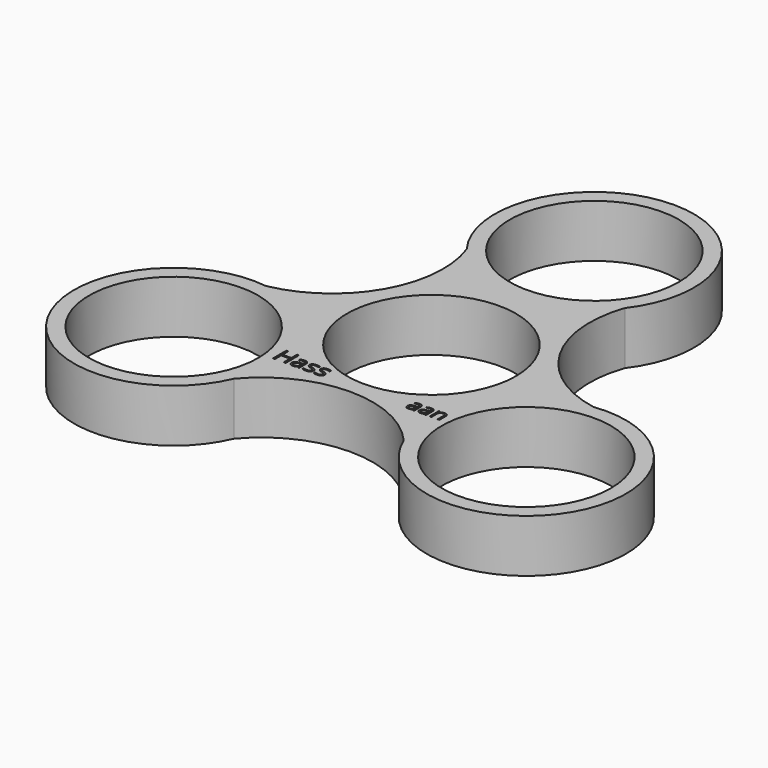
from build123d import *

# Parameters (mm, degrees)
F0_R         = 11.2
F1_DEPTH     = 7
F2_TEXT_SIZE = 3.0873436845
F3_DEPTH     = 0.51
F4_TEXT_SIZE = 2.8406800185
F5_DEPTH     = 0.64


# Not quite as in the source:
# - Text() gives the source's letters only with a copy of the font that has no kerning and outlines rounded to 1/6400 em; it was checked with that copy


with BuildPart() as f1:
    # F0 (on Top) → F1 (new body)
    with BuildSketch(Plane.XY):
        with BuildLine():
            ThreePointArc((21.7602352684, -0.3790794713), (11.6629101979, 6.6669216362), (10.4657940357, 18.9212685418))
            ThreePointArc((10.4657940357, 18.9212685418), (0.0710858988, 40.165152914), (-10.551825182, 19.0344562705))
            ThreePointArc((-10.551825182, 19.0344562705), (-11.605178601, 6.7669156953), (-21.6191962469, -0.3969907652))
            ThreePointArc((-21.6191962469, -0.3969907652), (-34.8195857199, -20.0210142628), (-11.2084100865, -18.6553767991))
            ThreePointArc((-11.2084100865, -18.6553767991), (-0.0577315969, -13.4338373316), (11.1534022111, -18.5242777766))
            ThreePointArc((11.1534022111, -18.5242777766), (34.748499821, -20.1441386512), (21.7602352684, -0.3790794713))
        make_face()
        with Locations((-23.352673207, -13.4826721624)):
            Circle(F0_R, mode=Mode.SUBTRACT)
        with Locations((23.352673207, -13.4826721624)):
            Circle(F0_R, mode=Mode.SUBTRACT)
        Circle(F0_R, mode=Mode.SUBTRACT)
        with Locations((0, 26.9653443247)):
            Circle(F0_R, mode=Mode.SUBTRACT)
    extrude(amount=F1_DEPTH)

    # F2 (on face) → F3 (cut)
    with BuildSketch(Plane.XY.offset(7)):
        with Locations((-11.2112455724, -12.6004500012)):
            Text('Hass', F2_TEXT_SIZE, font='Open Sans', text_align=(TextAlign.LEFT, TextAlign.BOTTOM))
    extrude(amount=-F3_DEPTH, mode=Mode.SUBTRACT)

    # F4 (on face) → F5 (cut)
    with BuildSketch(Plane.XY.offset(7)):
        with Locations((6.4620403573, -12.6233948395)):
            Text('aan', F4_TEXT_SIZE, font='Open Sans', text_align=(TextAlign.LEFT, TextAlign.BOTTOM))
    extrude(amount=-F5_DEPTH, mode=Mode.SUBTRACT)


solid = f1.part
